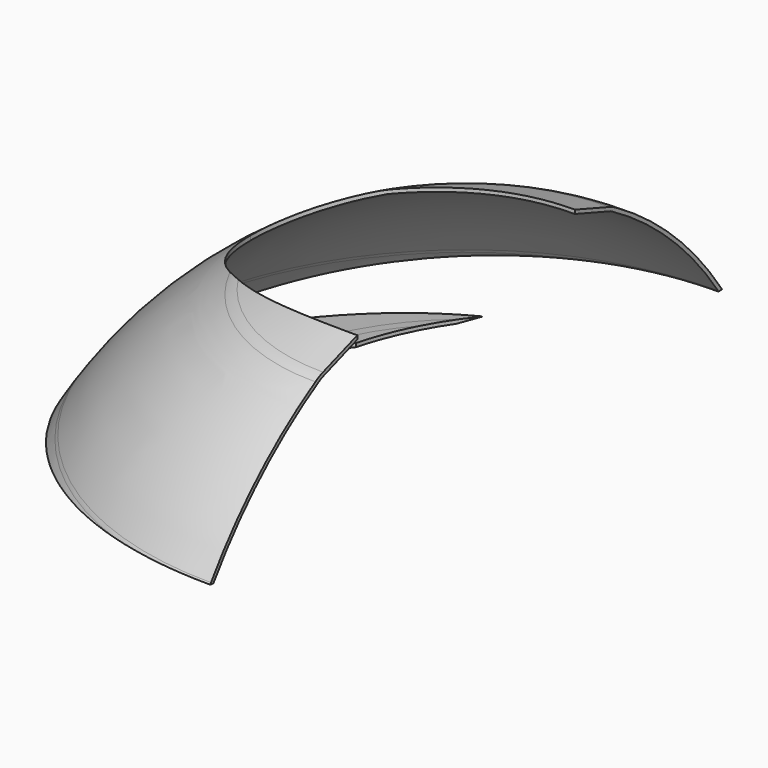
from build123d import *

# Parameters (mm, degrees)
F1_ANGLE = 180
F3_DEPTH = 16
F4_DEPTH = 10
F6_DEPTH = 100
F8_DEPTH = 120


# Not quite as in the source:
# - a feature names something its author has since deleted; it is built from what else it names


with BuildPart() as f1:
    # F0 (on Right) → F1 (revolve)
    with BuildSketch(Plane.YZ):
        with BuildLine():
            ThreePointArc((-55.3474134292, 7.6361638259), (-42.1679434739, 22.9837707191), (-25.8934941894, 35))
            Line((-25.8934941894, 35), (-27.4734756347, 35))
            ThreePointArc((-27.4734756347, 35), (-43.3676619435, 22.9550852631), (-56.2490525257, 7.7309299136))
            Line((-56.2490525257, 7.7309299136), (-55.3474134292, 7.6361638259))
        make_face()
        with BuildLine():
            Line((-27.4734756347, 35), (-25.8934941894, 35))
            Line((-25.8934941894, 35), (13.2809915289, 48.8023323047))
            Line((13.2809915289, 48.8023323047), (13.2809915289, 20.0909134001))
            Line((13.2809915289, 20.0909134001), (13.2809915289, 13.8023323047))
            Line((13.2809915289, 13.8023323047), (-32.3117841705, 5.2150216288))
            Line((-32.3117841705, 5.2150216288), (-29.5376830425, 4.9234518512))
            Line((-29.5376830425, 4.9234518512), (13.4290663861, 13.0161555837))
            Line((13.4290663861, 13.0161555837), (14.0809915289, 13.1389444171))
            Line((14.0809915289, 13.1389444171), (14.0809915289, 13.8023323047))
            Line((14.0809915289, 13.8023323047), (14.0809915289, 19.0225130607))
            Line((14.0809915289, 19.0225130607), (14.0809915289, 49.6023323047))
            Line((14.0809915289, 49.6023323047), (13.0151457916, 49.5568692779))
            Line((13.0151457916, 49.5568692779), (-25.3683284456, 36.0332337607))
            ThreePointArc((-25.3683284456, 36.0332337607), (-26.4512940518, 35.5785386451), (-27.4734756347, 35))
        make_face()
        with BuildLine():
            ThreePointArc((-60, 0), (-58.0031545142, 3.4887455953), (-55.8525170272, 6.8848457297))
            Line((-55.8525170272, 6.8848457297), (-56.7494178536, 6.9791138051))
            ThreePointArc((-56.7494178536, 6.9791138051), (-59.2223551886, 3.0035715179), (-61.4870824341, -1.0941554183))
            Line((-61.4870824341, -1.0941554183), (-59.8519251428, -0.786176721))
            Line((-59.8519251428, -0.786176721), (-53.878297587, 0.3389444171))
            Line((-53.878297587, 0.3389444171), (-32.2788666941, 4.407155239))
            Line((-32.2788666941, 4.407155239), (-35.052967822, 4.6987250166))
            Line((-35.052967822, 4.6987250166), (-60, 0))
        make_face()
        with BuildLine():
            ThreePointArc((-55.8525170272, 6.8848457297), (-55.6009099356, 7.2611398951), (-55.3474134292, 7.6361638259))
            Line((-55.3474134292, 7.6361638259), (-56.2490525257, 7.7309299136))
            ThreePointArc((-56.2490525257, 7.7309299136), (-56.500169896, 7.3556439459), (-56.7494178536, 6.9791138051))
            Line((-56.7494178536, 6.9791138051), (-55.8525170272, 6.8848457297))
        make_face()
        Polygon((-29.5376830425, 4.9234518512), (-32.3117841705, 5.2150216288), (-35.052967822, 4.6987250166), (-32.2788666941, 4.407155239), align=None)
    revolve(axis=Axis((0, 14.0809915289, 34.3124226827), (0, 0, -1)), revolution_arc=F1_ANGLE)

    # F2 (on Top) → F3 (cut)
    with BuildSketch(Plane.XY):
        with BuildLine():
            add(Edge.make_bspline(
                [(-40, 15), (-40, -129.8528137424), (28.2842712475, -27.4264068712), (96.5685424949, 75), (0, 75)],
                knots=[1.5707963268, 1.5707963268, 1.5707963268, 3.926990817, 3.926990817, 6.2831853072, 6.2831853072, 6.2831853072], degree=2, weights=[1, 0.3826834324, 1, 0.3826834324, 1]))
            add(Edge.make_bspline(
                [(0, 75), (-39.4701752826, 75), (-39.9964442864, 15.8)],
                knots=[0, 0, 0, 1.5574625984, 1.5574625984, 1.5574625984], degree=2, weights=[1, 0.7118052168, 1]))
            Line((-39.9964442864, 15.8), (0, 15.8))
            Line((0, 15.8), (0, 15))
            Line((0, 15), (-40, 15))
        make_face()
        with BuildLine():
            Line((0, 15.8), (-39.9964442864, 15.8))
            add(Edge.make_bspline(
                [(-39.9964442864, 15.8), (-40, 15.4000177794), (-40, 15)],
                knots=[1.5574625984, 1.5574625984, 1.5574625984, 1.5707963268, 1.5707963268, 1.5707963268], degree=2, weights=[1, 0.9999777765, 1]))
            Line((-40, 15), (0, 15))
            Line((0, 15), (0, 15.8))
        make_face()
    extrude(amount=F3_DEPTH, mode=Mode.SUBTRACT)

    # F2 (on Top) → F4 (cut)
    with BuildSketch(Plane.XY):
        with BuildLine():
            add(Edge.make_bspline(
                [(-40, 15), (-40, -129.8528137424), (28.2842712475, -27.4264068712), (96.5685424949, 75), (0, 75)],
                knots=[1.5707963268, 1.5707963268, 1.5707963268, 3.926990817, 3.926990817, 6.2831853072, 6.2831853072, 6.2831853072], degree=2, weights=[1, 0.3826834324, 1, 0.3826834324, 1]))
            add(Edge.make_bspline(
                [(0, 75), (-39.4701752826, 75), (-39.9964442864, 15.8)],
                knots=[0, 0, 0, 1.5574625984, 1.5574625984, 1.5574625984], degree=2, weights=[1, 0.7118052168, 1]))
            Line((-39.9964442864, 15.8), (0, 15.8))
            Line((0, 15.8), (0, 15))
            Line((0, 15), (-40, 15))
        make_face()
    extrude(amount=F4_DEPTH, mode=Mode.SUBTRACT)

    # F5 (on Top) → F6 (cut)
    with BuildSketch(Plane.XY):
        with BuildLine():
            add(Edge.make_bspline(
                [(-47.5, 14.081414789), (-47.5, -37.8801094381), (23.75, -11.8993473246), (95, 14.081414789), (23.75, 40.0621769025), (-47.5, 66.042939016), (-47.5, 14.081414789)],
                knots=[0, 0, 0, 2.0943951024, 2.0943951024, 4.1887902048, 4.1887902048, 6.2831853072, 6.2831853072, 6.2831853072], degree=2, weights=[1, 0.5, 1, 0.5, 1, 0.5, 1]))
        make_face()
    extrude(amount=F6_DEPTH, mode=Mode.SUBTRACT)

    # F7 (on Right) → F8 (cut)
    with BuildSketch(Plane.YZ):
        Polygon((94.4246426225, 0), (14, 0), (14, -1.5881112777), (94.696611166, -1.5881112777), align=None)
        Polygon((-66.4246426225, 0), (0, 0), (14, 0), (-58.0279476422, 7.5704423547), align=None)
        Polygon((86.0279476422, 7.5704423547), (14, 0), (94.4246426225, 0), align=None)
        Polygon((14, 0), (0, 0), (-66.4246426225, 0), (-66.696611166, -1.5881112777), (14, -1.5881112777), align=None)
    extrude(amount=-F8_DEPTH, mode=Mode.SUBTRACT)


solid = f1.part
